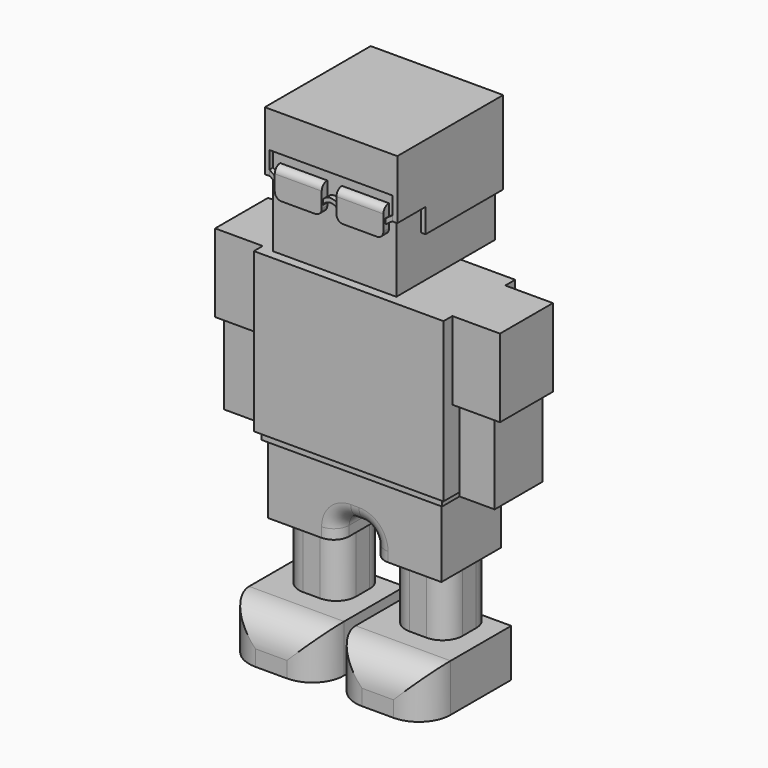
from build123d import *

# Parameters (mm, degrees)
F0_W           = 14.9648044608
F0_H           = 16.937578097
F0_W_2         = 1.812669565
F0_W_3         = 14.9648083382
F1_DEPTH       = 7.5
F2_DEPTH       = 14.2
F3_R           = 5
F4_W           = 8.966412507
F4_H           = 8.9642944624
F5_DEPTH       = 13.5
F5_DEPTH_BACK  = 4.3
F6_R           = 3.1384776311
F6_2_R         = 3.1384776311
F7_W           = 27.2792670876
F7_H           = 11.7013510317
F8_DEPTH       = 7.2
F9_W           = 10.8192516491
F9_H           = 11.7013510317
F10_DEPTH      = 3.7
F10_DEPTH_BACK = 2.3
F11_R          = 2.1727922061
F12_R          = 2.4142135624
F13_W          = 28.4332055598
F13_H          = 12.8980111331
F14_DEPTH      = 1.2
F15_W          = 29.8774708062
F15_H          = 14.1250584275
F15_W_2        = 28.4332055598
F15_H_2        = 12.8980111331
F16_DEPTH      = 25
F17_W          = 10.4226022959
F17_H          = 12.2977413476
F18_DEPTH      = 7.5
F18_DEPTH_BACK = 37.37747
F19_W          = 5.5065192282
F19_H          = 9.4299116172
F20_DEPTH      = 12.6
F21_W          = 10.0570814684
F21_H          = 9.5903184265
F22_DEPTH      = 2.8
F23_W          = 19.431643188
F23_H          = 19.43164
F23_W_2        = 10.0570814684
F23_H_2        = 9.5903184265
F24_DEPTH      = 19.43164
F26_DEPTH      = 12.5
F27_DEPTH      = 8.7
F25_W          = 19.431643188
F25_H          = 0.7098612483
F28_DEPTH      = 5.1
F29_DEPTH      = 0.6
F31_DEPTH      = 0.8
F32_DEPTH      = 1.1
F33_DEPTH      = 0.7
F34_R          = 1.0381118318


with BuildPart() as f1:
    # F0 (on Top) → F1 (new body)
    with BuildSketch(Plane.XY):
        with Locations((-8.3887370129, -8.4687890485)):
            Rectangle(F0_W, F0_H)
        with Locations((0, -8.4687890485)):
            Rectangle(F0_W_2, F0_H)
        with Locations((8.3887389516, -8.4687890485)):
            Rectangle(F0_W_3, F0_H)
    extrude(amount=F1_DEPTH)

    # F0 (on Top) → F2 (cut)
    with BuildSketch(Plane.XY):
        with Locations((0, -8.4687890485)):
            Rectangle(F0_W_2, F0_H)
    extrude(amount=F2_DEPTH, mode=Mode.SUBTRACT)

    # F3
    f3_edges = [f1.edges().sort_by_distance(p)[0] for p in [
        (-15.871139, -16.937578, 3.75),
        (-0.906335, -16.937578, 3.75),
        (0.906335, -16.937578, 3.75),
        (15.871143, -16.937578, 3.75),
        (-8.388737, -16.937578, 7.5),
        (8.388739, -16.937578, 7.5),
    ]]
    fillet(f3_edges, radius=F3_R)


with BuildPart() as f5:
    # F4 (on face) → F5 (new body, two sides)
    with BuildSketch(Plane.XY.offset(7.5)) as f5_sk:
        with Locations((-8.3887370129, -4.4944216307)):
            Rectangle(F4_W, F4_H)
    extrude(amount=F5_DEPTH)
    extrude(f5_sk.sketch, amount=-F5_DEPTH_BACK)

    # F6
    f6_edges = [f5.edges().sort_by_distance(p)[0] for p in [
        (-12.871943, -8.976569, 12.1),
        (-3.905531, -8.976569, 12.1),
        (-12.871943, -0.012274, 12.1),
        (-3.905531, -0.012274, 12.1),
    ]]
    fillet(f6_edges, radius=F6_R)


with BuildPart() as f5b:
    # F4 (on face) → F5, piece 2 (new body, two sides)
    with BuildSketch(Plane.XY.offset(7.5)) as f5_2_sk:
        with Locations((8.3887370129, -4.4944216307)):
            Rectangle(F4_W, F4_H)
    extrude(amount=F5_DEPTH)
    extrude(f5_2_sk.sketch, amount=-F5_DEPTH_BACK)

    # F6#2
    f6_2_edges = [f5b.edges().sort_by_distance(p)[0] for p in [
        (3.905531, -8.976569, 12.1),
        (12.871943, -8.976569, 12.1),
        (12.871943, -0.012274, 12.1),
        (3.905531, -0.012274, 12.1),
    ]]
    fillet(f6_2_edges, radius=F6_2_R)


with BuildPart() as f8:
    # F7 (on face) → F8 (new body)
    with BuildSketch(Plane.XY.offset(21)):
        with Locations((0, -5.1078274846)):
            Rectangle(F7_W, F7_H)
    extrude(amount=F8_DEPTH)

    # F9 (on face) → F10 (join, two sides)
    with BuildSketch(Plane(origin=(0, 0, 21), x_dir=(1, 0, 0), z_dir=(0, 0, -1))) as f10_sk:
        with Locations((-8.2300077192, 5.1078274846)):
            Rectangle(F9_W, F9_H)
        with Locations((8.2300077192, 5.1078274846)):
            Rectangle(F9_W, F9_H)
    extrude(amount=F10_DEPTH)
    extrude(f10_sk.sketch, amount=-F10_DEPTH_BACK)

    # F11
    f11_edges = [f8.edges().sort_by_distance(p)[0] for p in [
        (2.820382, -5.107827, 21),
        (-2.820382, -5.107827, 21),
    ]]
    fillet(f11_edges, radius=F11_R)

    # F12
    f12_edges = [f8.edges().sort_by_distance(p)[0] for p in [
        (2.183986, 0.742848, 20.363604),
        (-2.183986, -10.958503, 20.363604),
        (2.820382, -10.958503, 18.063604),
        (2.183986, -10.958503, 20.363604),
        (0, -10.958503, 21),
        (-2.820382, -10.958503, 18.063604),
        (2.820382, 0.742848, 18.063604),
        (0, 0.742848, 21),
        (-2.183986, 0.742848, 20.363604),
        (-2.820382, 0.742848, 18.063604),
    ]]
    fillet(f12_edges, radius=F12_R)

    # F13 (on face) → F14 (join)
    with BuildSketch(Plane.XY.offset(28.2)):
        with Locations((0, -5.1078274846)):
            Rectangle(F13_W, F13_H)
    extrude(amount=F14_DEPTH)


with BuildPart() as f16:
    # F15 (on face) → F16 (new body)
    with BuildSketch(Plane.XY.offset(29.4)):
        with Locations((0, -5.1078274846)):
            Rectangle(F15_W, F15_H)
        with Locations((0, -5.1078274846)):
            Rectangle(F15_W_2, F15_H_2, mode=Mode.SUBTRACT)
        with Locations((0, -5.1078274846)):
            Rectangle(F15_W_2, F15_H_2)
    extrude(amount=F16_DEPTH)

    # F17 (on face) → F18 (join, two sides)
    with BuildSketch(Plane(origin=(-14.9387354031, 0, 0), x_dir=(0, -1, 0), z_dir=(-1, 0, 0))) as f18_sk:
        with Locations((5.2113011479, 48.2511293262)):
            Rectangle(F17_W, F17_H)
    extrude(amount=F18_DEPTH)
    extrude(f18_sk.sketch, amount=-F18_DEPTH_BACK)


with BuildPart() as f20:
    # F19 (on face) → F20 (new body)
    with BuildSketch(Plane(origin=(0, 0, 42.1022586524), x_dir=(1, 0, 0), z_dir=(0, 0, -1))):
        with Locations((-18.5539349914, 5.3402557969)):
            Rectangle(F19_W, F19_H)
    extrude(amount=F20_DEPTH)


with BuildPart() as f20b:
    # F19 (on face) → F20, piece 2 (new body)
    with BuildSketch(Plane(origin=(0, 0, 42.1022586524), x_dir=(1, 0, 0), z_dir=(0, 0, -1))):
        with Locations((18.5539349914, 5.3402557969)):
            Rectangle(F19_W, F19_H)
    extrude(amount=F20_DEPTH)


with BuildPart() as f22:
    # F21 (on face) → F22 (new body)
    with BuildSketch(Plane.XY.offset(54.4)):
        with Locations((0, -5.2113011479)):
            Rectangle(F21_W, F21_H)
    extrude(amount=F22_DEPTH)

    # F23 (on face) → F24 (join)
    with BuildSketch(Plane.XY.offset(57.2)):
        with Locations((0, -5.2113011479)):
            Rectangle(F23_W, F23_H)
        with Locations((0, -5.2113011479)):
            Rectangle(F23_W_2, F23_H_2, mode=Mode.SUBTRACT)
        with Locations((0, -5.2113011479)):
            Rectangle(F23_W_2, F23_H_2)
    extrude(amount=F24_DEPTH)


with BuildPart() as f26:
    # F25 (on face) → F26 (new body)
    with BuildSketch(Plane.XY.offset(76.63164)):
        Polygon((9.715821594, -10.076250881), (10.4362731799, -10.076250881), (10.4362731799, 5.2143801004), (-10.4362731799, 5.2143801004), (-10.4362731799, -10.076250881), (-9.715821594, -10.076250881), (-9.715821594, 4.5045188521), (9.715821594, 4.5045188521), align=None)
    extrude(amount=-F26_DEPTH)

    # F25 (on face) → F27 (join)
    with BuildSketch(Plane.XY.offset(76.63164)):
        Polygon((-10.4362731799, -15.6369823962), (-9.715821594, -15.6369823962), (-9.715821594, -14.9271211479), (-9.715821594, -10.076250881), (-10.4362731799, -10.076250881), align=None)
        Polygon((9.715821594, -15.6369823962), (10.4362731799, -15.6369823962), (10.4362731799, -10.076250881), (9.715821594, -10.076250881), (9.715821594, -14.9271211479), align=None)
    extrude(amount=-F27_DEPTH)

    # F25 (on face) → F28 (join)
    with BuildSketch(Plane.XY.offset(76.63164)):
        with Locations((0, -15.2820517721)):
            Rectangle(F25_W, F25_H)
    extrude(amount=-F28_DEPTH)

    # F25 (on face) → F29 (join)
    with BuildSketch(Plane.XY.offset(76.63164)):
        Polygon((9.715821594, -10.076250881), (10.4362731799, -10.076250881), (10.4362731799, 5.2143801004), (-10.4362731799, 5.2143801004), (-10.4362731799, -10.076250881), (-9.715821594, -10.076250881), (-9.715821594, 4.5045188521), (9.715821594, 4.5045188521), align=None)
        Polygon((-10.4362731799, -15.6369823962), (-9.715821594, -15.6369823962), (-9.715821594, -14.9271211479), (-9.715821594, -10.076250881), (-10.4362731799, -10.076250881), align=None)
        with Locations((0, -15.2820517721)):
            Rectangle(F25_W, F25_H)
        Polygon((-9.715821594, -14.9271211479), (9.715821594, -14.9271211479), (9.715821594, -10.076250881), (9.715821594, 4.5045188521), (-9.715821594, 4.5045188521), (-9.715821594, -10.076250881), align=None)
        Polygon((9.715821594, -15.6369823962), (10.4362731799, -15.6369823962), (10.4362731799, -10.076250881), (9.715821594, -10.076250881), (9.715821594, -14.9271211479), align=None)
    extrude(amount=F29_DEPTH)


with BuildPart() as f31:
    # F30 (on face) → F31 (new body)
    with BuildSketch(Plane.XZ.offset(14.9271211479)):
        with BuildLine():
            Line((-1.1596926488, 67.5404071808), (-1.1596926488, 66.7473971844))
            ThreePointArc((-1.1596926488, 66.7473971844), (0.0084986196, 67.4038543011), (1.1596926488, 66.7180269957))
            Line((1.1596926488, 66.7180269957), (1.1596926488, 67.5404071808))
            ThreePointArc((1.1596926488, 67.5404071808), (0, 68.070335216), (-1.1596926488, 67.5404071808))
        make_face()
    extrude(amount=F31_DEPTH)

    # F30 (on face) → F32 (join)
    with BuildSketch(Plane.XZ.offset(14.9271211479)):
        Polygon((1.1596926488, 67.5404071808), (1.1596926488, 66.7180269957), (1.1596926488, 65.278865397), (8.561090799, 65.278865397), (8.561090799, 67.1585947275), (8.561090799, 67.9809674621), (8.561090799, 69.8019489646), (1.1596926488, 69.8019489646), align=None)
        Polygon((-8.561090799, 65.278865397), (-1.1596926488, 65.278865397), (-1.1596926488, 66.7473971844), (-1.1596926488, 67.5404071808), (-1.1596926488, 69.8019489646), (-8.561090799, 69.8019489646), (-8.561090799, 67.9809674621), (-8.561090799, 67.1585947275), align=None)
    extrude(amount=F32_DEPTH)

    # F30 (on face) → F33 (join)
    with BuildSketch(Plane.XZ.offset(14.9271211479)):
        Polygon((-9.715821594, 67.9809674621), (-8.561090799, 67.1585947275), (-8.561090799, 67.9809674621), (-9.715821594, 68.8033401966), align=None)
        Polygon((8.561090799, 67.9809674621), (8.561090799, 67.1585947275), (9.715821594, 67.9809674621), (9.715821594, 68.8033401966), align=None)
    extrude(amount=F33_DEPTH)

    # F34
    f34_edges = [f31.edges().sort_by_distance(p)[0] for p in [
        (-1.159693, -15.477121, 65.278865),
        (-8.561091, -15.477121, 65.278865),
        (1.159693, -15.477121, 65.278865),
        (8.561091, -15.477121, 65.278865),
        (-4.860392, -16.027121, 69.801949),
        (4.860392, -16.027121, 69.801949),
    ]]
    fillet(f34_edges, radius=F34_R)


solid = Compound([f1.part, f5.part, f5b.part, f8.part, f16.part, f20.part, f20b.part, f22.part, f26.part, f31.part])
